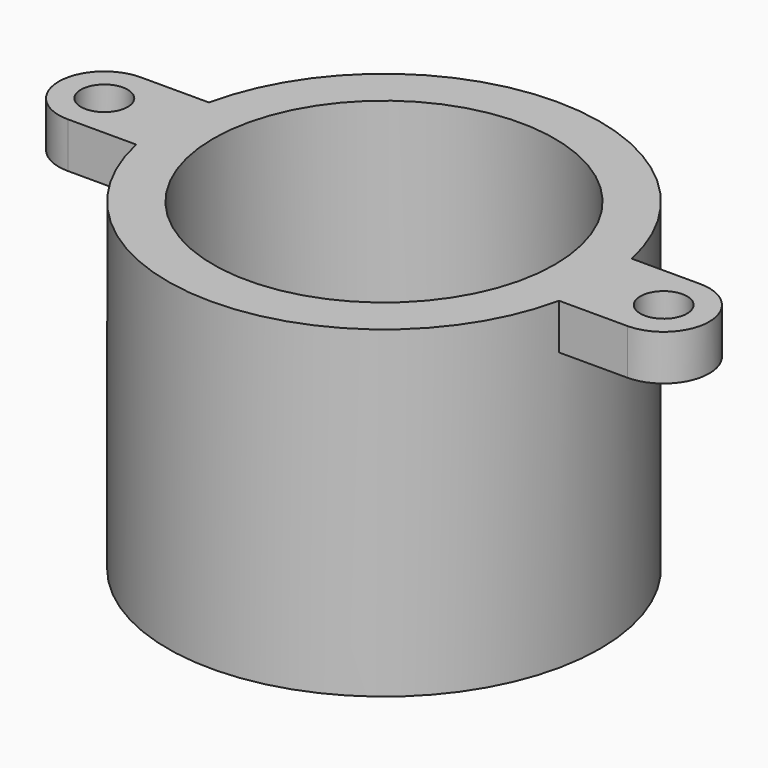
from build123d import *

# Parameters (mm, degrees)
F0_R     = 15.08125
F0_R_2   = 11.90625
F1_DEPTH = 22.5425
F2_R     = 1.63195
F3_DEPTH = 3.175


# Not quite as in the source:
# - a pattern or mirror of a feature is missing from the dataset's text; its kind, count and spacing are read off the source's solid


with BuildPart() as f1:
    # F0 (on Top) → F1 (new body)
    with BuildSketch(Plane.XY):
        Circle(F0_R)
        Circle(F0_R_2, mode=Mode.SUBTRACT)
    extrude(amount=-F1_DEPTH)

    # F2 (on Top) → F3 (join)
    with BuildSketch(Plane.XY):
        with BuildLine():
            Line((19.5057518992, 3.175), (14.7432518992, 3.175))
            Line((14.7432518992, 3.175), (14.7432518992, -3.175))
            Line((14.7432518992, -3.175), (19.5057518992, -3.175))
            ThreePointArc((19.5057518992, -3.175), (22.6807518992, 0), (19.5057518992, 3.175))
        make_face()
        with Locations((19.5057518992, 0)):
            Circle(F2_R, mode=Mode.SUBTRACT)
    f3 = extrude(amount=-F3_DEPTH)

    # F3_copies: F3 across plane
    add(f3.mirror(Plane(origin=(0, 0, 0), x_dir=(0, 0, -1), z_dir=(-1, 0, 0))))


solid = f1.part
